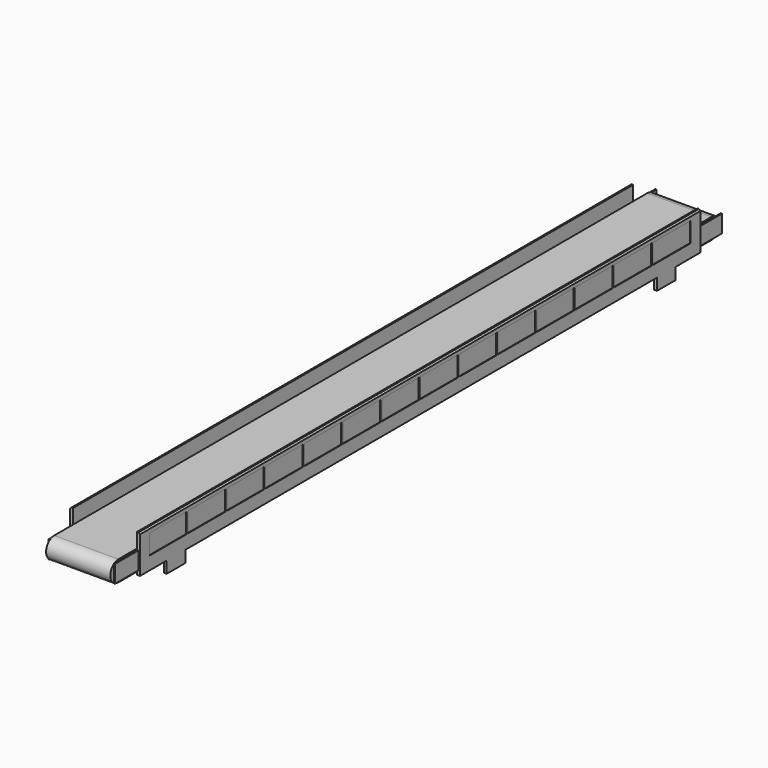
from build123d import *

# Parameters (mm, degrees)
F1_R          = 150
F2_DEPTH      = 1100
F4_DEPTH      = 1100
F6_START      = -400
F6_DEPTH      = 12000
F7_W          = 20
F7_H          = 300
F8_DEPTH      = 500
F8_DEPTH_BACK = 12500
F9_W          = 800
F9_H          = 340
F10_DEPTH     = 10
F11_W         = 800
F11_H         = 340
F12_DEPTH     = 10
F13_W         = 50
F13_H         = 400
F14_DEPTH     = 200


with BuildPart() as f2:
    # F1 (on Right) → F2 (new body)
    with BuildSketch(Plane.YZ):
        Circle(F1_R)
    extrude(amount=F2_DEPTH)


with BuildPart() as f2b:
    # F1 (on Right) → F2, piece 2 (new body)
    with BuildSketch(Plane.YZ):
        with Locations((12700, 0)):
            Circle(F1_R)
    extrude(amount=F2_DEPTH)


with BuildPart() as f4:
    # F3 (on face) → F4 (new body)
    with BuildSketch(Plane.YZ.offset(1100)):
        with BuildLine():
            ThreePointArc((0, -175), (123.7436867076, -123.7436867076), (175, 0))
            ThreePointArc((175, 0), (123.7436867076, 123.7436867076), (0, 175))
            Line((0, 175), (0, -175))
        make_face()
        with BuildLine():
            ThreePointArc((0, 175), (123.7436867076, 123.7436867076), (175, 0))
            ThreePointArc((175, 0), (123.7436867076, -123.7436867076), (0, -175))
            Line((0, -175), (12700, -175))
            ThreePointArc((12700, -175), (12525, 0), (12700, 175))
            Line((12700, 175), (0, 175))
        make_face()
        with BuildLine():
            Line((0, -175), (0, 175))
            ThreePointArc((0, 175), (-175, 0), (0, -175))
        make_face()
        with BuildLine():
            Line((12700, -175), (12700, 175))
            ThreePointArc((12700, 175), (12525, 0), (12700, -175))
        make_face()
        with BuildLine():
            ThreePointArc((12875, 0), (12823.7436867076, 123.7436867076), (12700, 175))
            Line((12700, 175), (12700, -175))
            ThreePointArc((12700, -175), (12823.7436867076, -123.7436867076), (12875, 0))
        make_face()
    extrude(amount=-F4_DEPTH)


with BuildPart() as f6:
    # F5 (on Front) → F6 (new body)
    with BuildSketch(Plane.XZ.offset(F6_START)):
        Polygon((0, -225), (0, 425), (-25, 425), (-50, 401.8485546112), (-50, -225), align=None)
    extrude(amount=-F6_DEPTH)

    # F7 (on face) → F8 (join, two sides)
    with BuildSketch(Plane.XZ.offset(-400)) as f8_sk:
        with Locations((-10, 0)):
            Rectangle(F7_W, F7_H)
    extrude(amount=F8_DEPTH)
    extrude(f8_sk.sketch, amount=-F8_DEPTH_BACK)

    # F9 (on face) → F10 (cut)
    with BuildSketch(Plane(origin=(-50, 0, 0), x_dir=(0, -1, 0), z_dir=(-1, 0, 0))):
        with Locations((-1000, 170)):
            Rectangle(F9_W, F9_H)
        with Locations((-1830, 170)):
            Rectangle(F9_W, F9_H)
        with Locations((-2660, 170)):
            Rectangle(F9_W, F9_H)
        with Locations((-3490, 170)):
            Rectangle(F9_W, F9_H)
        with Locations((-4320, 170)):
            Rectangle(F9_W, F9_H)
        with Locations((-5150, 170)):
            Rectangle(F9_W, F9_H)
        with Locations((-5980, 170)):
            Rectangle(F9_W, F9_H)
        with Locations((-6810, 170)):
            Rectangle(F9_W, F9_H)
        with Locations((-7640, 170)):
            Rectangle(F9_W, F9_H)
        with Locations((-8470, 170)):
            Rectangle(F9_W, F9_H)
        with Locations((-9300, 170)):
            Rectangle(F9_W, F9_H)
        with Locations((-10130, 170)):
            Rectangle(F9_W, F9_H)
        with Locations((-10960, 170)):
            Rectangle(F9_W, F9_H)
        with Locations((-11790, 170)):
            Rectangle(F9_W, F9_H)
    extrude(amount=-F10_DEPTH, mode=Mode.SUBTRACT)

    # F13 (on face) → F14, piece 2 (join)
    with BuildSketch(Plane(origin=(0, 0, -225), x_dir=(1, 0, 0), z_dir=(0, 0, -1))):
        with Locations((-25, -1171.534705162)):
            Rectangle(F13_W, F13_H)
        with Locations((-25, -11671.534705162)):
            Rectangle(F13_W, F13_H)
    extrude(amount=F14_DEPTH)


with BuildPart() as f6b:
    # F5 (on Front) → F6, piece 2 (new body)
    with BuildSketch(Plane.XZ.offset(F6_START)):
        Polygon((1125, 425), (1100, 425), (1100, -225), (1150, -225), (1150, 401.8485546112), align=None)
    extrude(amount=-F6_DEPTH)

    # F7 (on face) → F8, piece 2 (join, two sides)
    with BuildSketch(Plane.XZ.offset(-400)) as f8_2_sk:
        with Locations((1110, 0)):
            Rectangle(F7_W, F7_H)
    extrude(amount=F8_DEPTH)
    extrude(f8_2_sk.sketch, amount=-F8_DEPTH_BACK)

    # F11 (on face) → F12 (cut)
    with BuildSketch(Plane.YZ.offset(1150)):
        with Locations((1000, 170)):
            Rectangle(F11_W, F11_H)
        with Locations((1830, 170)):
            Rectangle(F11_W, F11_H)
        with Locations((2660, 170)):
            Rectangle(F11_W, F11_H)
        with Locations((3490, 170)):
            Rectangle(F11_W, F11_H)
        with Locations((4320, 170)):
            Rectangle(F11_W, F11_H)
        with Locations((5150, 170)):
            Rectangle(F11_W, F11_H)
        with Locations((5980, 170)):
            Rectangle(F11_W, F11_H)
        with Locations((6810, 170)):
            Rectangle(F11_W, F11_H)
        with Locations((7640, 170)):
            Rectangle(F11_W, F11_H)
        with Locations((8470, 170)):
            Rectangle(F11_W, F11_H)
        with Locations((9300, 170)):
            Rectangle(F11_W, F11_H)
        with Locations((10130, 170)):
            Rectangle(F11_W, F11_H)
        with Locations((10960, 170)):
            Rectangle(F11_W, F11_H)
        with Locations((11790, 170)):
            Rectangle(F11_W, F11_H)
    extrude(amount=-F12_DEPTH, mode=Mode.SUBTRACT)

    # F13 (on face) → F14 (join)
    with BuildSketch(Plane(origin=(0, 0, -225), x_dir=(1, 0, 0), z_dir=(0, 0, -1))):
        with Locations((1125, -1171.534705162)):
            Rectangle(F13_W, F13_H)
        with Locations((1125, -11671.534705162)):
            Rectangle(F13_W, F13_H)
    extrude(amount=F14_DEPTH)


solid = Compound([f2.part, f2b.part, f4.part, f6.part, f6b.part])
